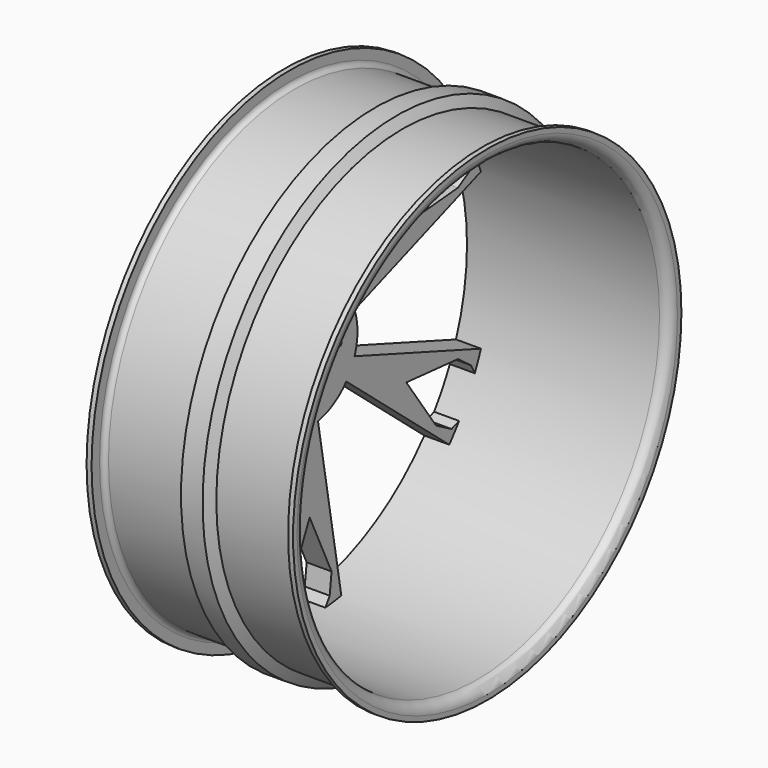
from build123d import *

# Parameters (mm, degrees)
F2_R     = 3.1146523594
F2_R_2   = 22.9197931693
F3_DEPTH = 25
F4_COUNT = 6
F5_DEPTH = 25


# Not quite as in the source:
# - a feature names something its author has since deleted; it is built from what else it names


with BuildPart() as f1:
    # F0 (on Top) → F1 (revolve)
    with BuildSketch(Plane.XY):
        with BuildLine():
            Line((-79.7097083151, 53.5523933172), (-79.7097083151, 33.5523933172))
            Line((-79.7097083151, 33.5523933172), (113.4902916849, 33.5523933172))
            ThreePointArc((113.4902916849, 33.5523933172), (120.5613594967, 36.4813255054), (123.4902916849, 43.5523933172))
            Line((123.4902916849, 43.5523933172), (123.4902916849, 48.5523933172))
            Line((123.4902916849, 48.5523933172), (118.4902916849, 48.5523933172))
            Line((118.4902916849, 48.5523933172), (118.4902916849, 43.5523933172))
            ThreePointArc((118.4902916849, 43.5523933172), (117.0258255908, 40.0168594113), (113.4902916849, 38.5523933172))
            Line((113.4902916849, 38.5523933172), (38.4902916849, 38.5523933172))
            Line((38.4902916849, 38.5523933172), (5.2902916849, 38.5523933172))
            Line((5.2902916849, 38.5523933172), (-69.7097083151, 38.5523933172))
            ThreePointArc((-69.7097083151, 38.5523933172), (-73.2452422211, 40.0168594113), (-74.7097083151, 43.5523933172))
            Line((-74.7097083151, 43.5523933172), (-74.7097083151, 53.5523933172))
            Line((-74.7097083151, 53.5523933172), (-79.7097083151, 53.5523933172))
        make_face()
        Polygon((11.0637943768, 48.5523933172), (5.2902916849, 38.5523933172), (38.4902916849, 38.5523933172), (32.716788993, 48.5523933172), align=None)
    revolve(axis=Axis((21.8902916849, -195.0476066828, 0), (1, 0, 0)))

    # F2 (on face) → F3 (join)
    with BuildSketch(Plane(origin=(-79.7097083151, 0, 0), x_dir=(0, -1, 0), z_dir=(-1, 0, 0))):
        with BuildLine():
            ThreePointArc((184.6287160228, 59.0884651807), (189.8182621179, 59.7716818855), (195.0476066828, 60))
            Line((195.0476066828, 60), (195.0476066828, 139.9987626345))
            Line((195.0476066828, 139.9987626345), (167.5774196696, 198.9087687919))
            Line((167.5774196696, 198.9087687919), (167.7933331286, 221.202246743))
            Line((167.7933331286, 221.202246743), (175.3516332681, 227.7499256449))
            ThreePointArc((175.3516332681, 227.7499256449), (165.3226894728, 226.6591919532), (155.3516332681, 225.1270523386))
            Line((155.3516332681, 225.1270523386), (184.6287160228, 59.0884651807))
        make_face()
        with BuildLine():
            Line((195.0476066828, 139.9987626345), (195.0476066828, 60))
            ThreePointArc((195.0476066828, 60), (200.2769512476, 59.7716818855), (205.4664973428, 59.0884651807))
            Line((205.4664973428, 59.0884651807), (234.7435800974, 225.1270523386))
            ThreePointArc((234.7435800974, 225.1270523386), (224.7725238927, 226.6591919532), (214.7435800974, 227.7499256449))
            Line((214.7435800974, 227.7499256449), (220.1414219841, 219.3318912564))
            Line((220.1414219841, 219.3318912564), (222.5177936959, 198.9087687919))
            Line((222.5177936959, 198.9087687919), (195.0476066828, 139.9987626345))
        make_face()
        with BuildLine():
            ThreePointArc((205.4664973428, 59.0884651807), (200.2769512476, 59.7716818855), (195.0476066828, 60))
            ThreePointArc((195.0476066828, 60), (189.8182621179, 59.7716818855), (184.6287160228, 59.0884651807))
            ThreePointArc((184.6287160228, 59.0884651807), (156.4803501016, -45.9626665871), (255.0476066828, 0))
            ThreePointArc((255.0476066828, 0), (241.0102732699, 38.5672565812), (205.4664973428, 59.0884651807))
        make_face()
        with Locations((158.1552479456, -1.5052259386)):
            Circle(F2_R, mode=Mode.SUBTRACT)
        with Locations((185.0787958079, -35.5518585739)):
            Circle(F2_R, mode=Mode.SUBTRACT)
        with Locations((195.0476066828, 0)):
            Circle(F2_R_2, mode=Mode.SUBTRACT)
        with Locations((225.7789014718, -20.4670310233)):
            Circle(F2_R, mode=Mode.SUBTRACT)
        with Locations((224.0094022556, 22.9025377527)):
            Circle(F2_R, mode=Mode.SUBTRACT)
        with Locations((182.215685933, 34.6215777831)):
            Circle(F2_R, mode=Mode.SUBTRACT)
    extrude(amount=-F3_DEPTH)

    # F4: F1 ×6 about axis
    f4_axis = Axis((21.8902916849, -195.0476066828, 0), (1, 0, 0))


with BuildPart() as f1_1:
    add(f1.part)
    for i in range(1, F4_COUNT):
        add(f1.part.rotate(f4_axis, i * 360 / F4_COUNT))

    # F2 (on face) → F5 (cut)
    with BuildSketch(Plane(origin=(-79.7097083151, 0, 0), x_dir=(0, -1, 0), z_dir=(-1, 0, 0))):
        with Locations((158.1552479456, -1.5052259386)):
            Circle(F2_R)
        with Locations((182.215685933, 34.6215777831)):
            Circle(F2_R)
        with Locations((224.0094022556, 22.9025377527)):
            Circle(F2_R)
        with Locations((225.7789014718, -20.4670310233)):
            Circle(F2_R)
        with Locations((185.0787958079, -35.5518585739)):
            Circle(F2_R)
        with Locations((195.0476066828, 0)):
            Circle(F2_R_2)
    extrude(amount=-F5_DEPTH, mode=Mode.SUBTRACT)


solid = f1_1.part
